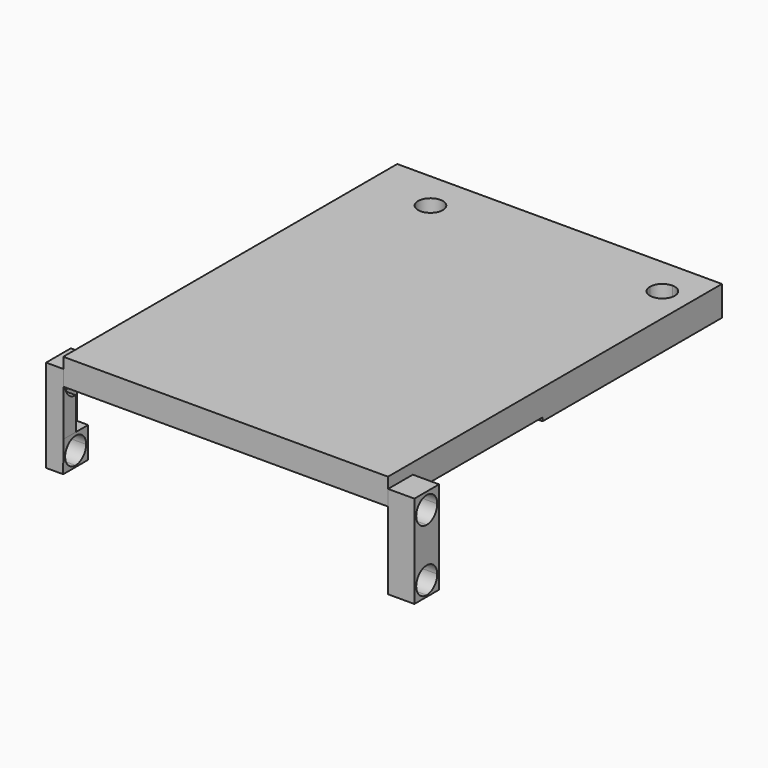
from build123d import *

# Parameters (mm, degrees)
F1_DEPTH  = 3.4
F2_R      = 1.6
F2_W      = 2
F2_H      = 5
F3_DEPTH  = 9.4
F4_DEPTH  = 44.24
F5_W      = 43.4320680797
F5_H      = 5.540763028
F6_DEPTH  = 55
F7_W      = 42
F7_H      = 6
F8_DEPTH  = 25
F9_D      = 3.4
F11_DEPTH = 25


# Not quite as in the source:
# - after a boolean that leaves OpenCascade's solid faulty, fix() repairs it
# - a feature names something its author has since deleted; it is built from what else it names


with BuildPart() as f1:
    # F0 (on Right) → F1 (new body)
    with BuildSketch(Plane.YZ):
        Polygon((0, 4), (-2, 4), (-2, -4), (0, -4), (2, -4), (2, 4), align=None)
        with BuildLine():
            ThreePointArc((1.7, -2.1), (1.202081528, -3.302081528), (0, -3.8))
            ThreePointArc((0, -3.8), (-1.202081528, -0.897918472), (1.7, -2.1))
        make_face(mode=Mode.SUBTRACT)
        Polygon((-2, 8), (-2, 4), (0, 4), (2, 4), (2, 8), align=None)
        with BuildLine():
            ThreePointArc((1.7, 5.9), (1.202081528, 4.697918472), (0, 4.2))
            ThreePointArc((0, 4.2), (-1.202081528, 7.102081528), (1.7, 5.9))
        make_face(mode=Mode.SUBTRACT)
    extrude(amount=F1_DEPTH)

    # F2 (on Top) → F3 (join)
    with BuildSketch(Plane.XY):
        with BuildLine():
            Line((-42, -2.019777894), (0, -2.019777894))
            Line((0, -2.019777894), (0, 1.980222106))
            Line((0, 1.980222106), (0, 46.980222106))
            Line((0, 46.980222106), (-2, 46.980222106))
            Line((-2, 46.980222106), (-2.1, 46.980222106))
            ThreePointArc((-2.1, 46.980222106), (-3.7, 45.380222106), (-5.3, 46.980222106))
            ThreePointArc((-5.3, 46.980222106), (-4.8313708499, 48.1115929559), (-3.7, 48.580222106))
            Line((-3.7, 48.580222106), (-3.7, 51.980222106))
            Line((-3.7, 51.980222106), (-42, 51.980222106))
            Line((-42, 51.980222106), (-42, 1.980222106))
            Line((-42, 1.980222106), (-42, -2.019777894))
        make_face()
        with Locations((-33.7, 46.980222106)):
            Circle(F2_R, mode=Mode.SUBTRACT)
        with BuildLine():
            Line((-2.1, 46.980222106), (-2, 46.980222106))
            Line((-2, 46.980222106), (-2, 51.980222106))
            Line((-2, 51.980222106), (-3.7, 51.980222106))
            Line((-3.7, 51.980222106), (-3.7, 48.580222106))
            ThreePointArc((-3.7, 48.580222106), (-2.5686291501, 48.1115929559), (-2.1, 46.980222106))
        make_face()
        with Locations((-1, 49.480222106)):
            Rectangle(F2_W, F2_H)
    extrude(amount=F3_DEPTH)

    # F0 (on Right) → F4 (join)
    with BuildSketch(Plane.YZ):
        Polygon((0, 4), (-2, 4), (-2, -4), (0, -4), (2, -4), (2, 4), align=None)
        with BuildLine():
            ThreePointArc((1.7, -2.1), (1.202081528, -3.302081528), (0, -3.8))
            ThreePointArc((0, -3.8), (-1.202081528, -0.897918472), (1.7, -2.1))
        make_face(mode=Mode.SUBTRACT)
        Polygon((-2, 8), (-2, 4), (0, 4), (2, 4), (2, 8), align=None)
        with BuildLine():
            ThreePointArc((1.7, 5.9), (1.202081528, 4.697918472), (0, 4.2))
            ThreePointArc((0, 4.2), (-1.202081528, 7.102081528), (1.7, 5.9))
        make_face(mode=Mode.SUBTRACT)
    extrude(amount=-F4_DEPTH)

    # F5 (on Front) → F6 (cut)
    with BuildSketch(Plane.XZ):
        with Locations((-21.7160340399, 2.770381514)):
            Rectangle(F5_W, F5_H)
    extrude(amount=-F6_DEPTH, mode=Mode.SUBTRACT)

    # F7 (on face) → F8 (cut)
    with BuildSketch(Plane.XZ.offset(2.019777894)):
        with Locations((-21, 3)):
            Rectangle(F7_W, F7_H)
    extrude(amount=-F8_DEPTH, mode=Mode.SUBTRACT)

    # F9 (through all)
    with Locations(Plane.YZ):
        with Locations((0, 5.9)):
            Hole(F9_D / 2)

    # F10 (on face) → F11 (cut)
    with BuildSketch(Plane.XZ.offset(2)):
        Polygon((0, -4), (0, 0), (-42, 0), (-42.0278720558, -4), align=None)
    extrude(amount=-F11_DEPTH, mode=Mode.SUBTRACT)

    add(f1.part.fix(), mode=Mode.REPLACE)


solid = f1.part
